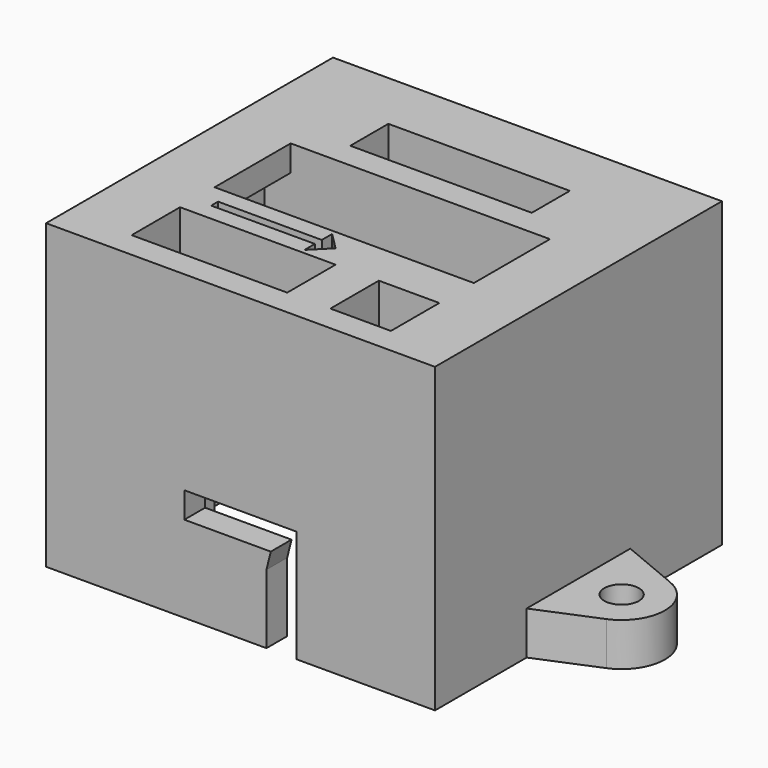
from build123d import *

# Parameters (mm, degrees)
F0_W      = 45
F0_H      = 41.5
F0_W_2    = 18
F0_H_2    = 4
F0_W_3    = 7
F0_H_3    = 3
F0_W_4    = 30
F0_H_4    = 11
F0_W_5    = 8
F0_H_5    = 3.5
F1_DEPTH  = 35
F2_W      = 21
F2_H      = 5.5
F3_DEPTH  = 4
F4_R      = 1.75
F5_DEPTH  = 25
F7_DEPTH  = 4
F9_START  = -8
F8_R      = 3.25
F9_DEPTH  = 17
F11_START = -3
F10_W     = 36
F10_H     = 11
F11_DEPTH = 32.001
F12_W     = 18
F12_H     = 7
F13_DEPTH = 4.5
F14_W     = 7
F14_H     = 4
F15_DEPTH = 3.5
F17_START = -20
F16_W     = 30
F16_H     = 12.5
F16_H_2   = 12
F17_DEPTH = 15.001
F19_DEPTH = 2
F20_R     = 2
F21_DEPTH = 5
F23_DEPTH = 10
F24_SIZE  = 0.74999


# Not quite as in the source:
# - a fillet or chamfer is up to 0.001 mm smaller than in the source, because OpenCascade refuses the exact size


with BuildPart() as f1:
    # F0 (on Top) → F1 (new body)
    with BuildSketch(Plane.XY):
        Rectangle(F0_W, F0_H)
        with Locations((-6, -12.75)):
            Rectangle(F0_W_2, F0_H_2, mode=Mode.SUBTRACT)
        with Locations((11.5, -12.25)):
            Rectangle(F0_W_3, F0_H_3, mode=Mode.SUBTRACT)
        with Locations((0, -0.25)):
            Rectangle(F0_W_4, F0_H_4, mode=Mode.SUBTRACT)
        with Locations((-4.75, 12)):
            Rectangle(F0_W_5, F0_H_5, mode=Mode.SUBTRACT)
        with Locations((4.75, 12)):
            Rectangle(F0_W_5, F0_H_5, mode=Mode.SUBTRACT)
    extrude(amount=F1_DEPTH)

    # F2 (on face) → F3 (cut)
    with BuildSketch(Plane.XY.offset(35)):
        with Locations((0, 11)):
            Rectangle(F2_W, F2_H)
    extrude(amount=-F3_DEPTH, mode=Mode.SUBTRACT)

    # F4 (on face) → F5 (cut)
    with BuildSketch(Plane.XZ.offset(-13.75)):
        with Locations((4.75, 23.5)):
            Circle(F4_R)
        with Locations((-4.75, 23.5)):
            Circle(F4_R)
    extrude(amount=-F5_DEPTH, mode=Mode.SUBTRACT)

    # F6 (on face) → F7 (cut)
    with BuildSketch(Plane.XZ.offset(-13.75)):
        Polygon((4.75, 26.9641016151), (1.75, 25.2320508076), (1.75, 21.7679491924), (1.75, -5.2918036282), (7.75, -5.2918036282), (7.75, 21.7679491924), (7.75, 25.2320508076), align=None)
        Polygon((-1.75, 21.7679491924), (-1.75, 25.2320508076), (-4.75, 26.9641016151), (-7.75, 25.2320508076), (-7.75, 21.7679491924), (-7.75, -5.2918036282), (-1.75, -5.2918036282), align=None)
    extrude(amount=-F7_DEPTH, mode=Mode.SUBTRACT)

    # F8 (on face) → F9 (cut)
    with BuildSketch(Plane.XY.offset(31).offset(F9_START)):
        with Locations((4.75, 12)):
            Circle(F8_R)
        with Locations((-4.75, 12)):
            Circle(F8_R)
    extrude(amount=-F9_DEPTH, mode=Mode.SUBTRACT)

    # F10 (on face) → F11 (cut)
    with BuildSketch(Plane.XY.offset(35).offset(F11_START)):
        with Locations((0, -0.25)):
            Rectangle(F10_W, F10_H)
    extrude(amount=-F11_DEPTH, mode=Mode.SUBTRACT)

    # F12 (on face) → F13 (cut)
    with BuildSketch(Plane.XY.offset(35)):
        with Locations((-6, -14.25)):
            Rectangle(F12_W, F12_H)
    extrude(amount=-F13_DEPTH, mode=Mode.SUBTRACT)

    # F14 (on face) → F15 (cut)
    with BuildSketch(Plane.XY.offset(35)):
        with Locations((11.5, -15.75)):
            Rectangle(F14_W, F14_H)
    extrude(amount=-F15_DEPTH, mode=Mode.SUBTRACT)

    # F16 (on face) → F17 (cut)
    with BuildSketch(Plane.XY.offset(35).offset(F17_START)):
        with Locations((0, 11.5)):
            Rectangle(F16_W, F16_H)
        with Locations((0, -11.75)):
            Rectangle(F16_W, F16_H_2)
    extrude(amount=-F17_DEPTH, mode=Mode.SUBTRACT)

    # F18 (on face) → F19 (cut)
    with BuildSketch(Plane.XY.offset(35)):
        Polygon((-1, -7.75), (-13, -7.75), (-13, -8.75), (-1, -8.75), (-1, -10.25), (1, -8.25), (-1, -6.25), align=None)
    extrude(amount=-F19_DEPTH, mode=Mode.SUBTRACT)

    # F20 (on Top) → F21 (join)
    with BuildSketch(Plane.XY):
        with BuildLine():
            Line((22.5, -7.5), (29.4230769231, -4.6153846154))
            ThreePointArc((29.4230769231, -4.6153846154), (32.5, 0), (29.4230769231, 4.6153846154))
            Line((29.4230769231, 4.6153846154), (22.5, 7.5))
            Line((22.5, 7.5), (22.5, -7.5))
        make_face()
        with Locations((27.5, 0)):
            Circle(F20_R, mode=Mode.SUBTRACT)
        with BuildLine():
            Line((-29.4230769231, -4.6153846154), (-22.5, -7.5))
            Line((-22.5, -7.5), (-22.5, 7.5))
            Line((-22.5, 7.5), (-29.4230769231, 4.6153846154))
            ThreePointArc((-29.4230769231, 4.6153846154), (-32.5, 0), (-29.4230769231, -4.6153846154))
        make_face()
        with Locations((-27.5, 0)):
            Circle(F20_R, mode=Mode.SUBTRACT)
    extrude(amount=F21_DEPTH)

    # F22 (on face) → F23 (cut)
    with BuildSketch(Plane.XZ.offset(20.75)):
        Polygon((3, 8), (3, 0), (6.5, 0), (6.5, 13), (-6.5, 13), (-6.5, 10), (3.5, 10), align=None)
    extrude(amount=-F23_DEPTH, mode=Mode.SUBTRACT)

    # F24 (size 0.75 in the source; OpenCascade refuses exactly that, so slightly less here)
    f24_edges = [f1.edges().sort_by_distance(p)[0] for p in [
        (-7.75, 15.75, 15),
        (-4.75, 8.75, 15),
        (8.119306, 10.25, 15),
        (1.380694, 10.25, 15),
        (-1.380694, 10.25, 15),
        (-8.119306, 10.25, 15),
        (-8.75, 12, 15),
        (-8.25, 13.75, 15),
        (-1.25, 13.75, 15),
        (1.25, 13.75, 15),
        (8.25, 13.75, 15),
        (-1.75, 15.75, 15),
        (1.75, 15.75, 15),
        (4.75, 8.75, 15),
        (8.75, 12, 15),
        (7.75, 15.75, 15),
        (-0.75, 12, 15),
        (0.75, 12, 15),
        (4.75, 10.25, 23),
        (-4.75, 10.25, 23),
    ]]
    chamfer(f24_edges, length=F24_SIZE)


solid = f1.part
